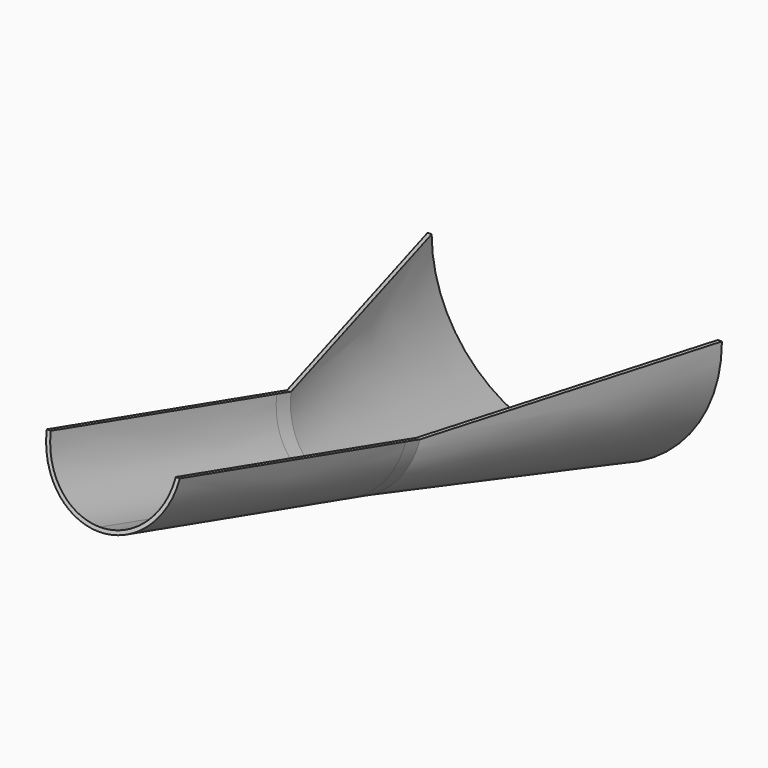
from build123d import *

# Parameters (mm, degrees)
F1_ANGLE      = 180
F3_DEPTH      = 44.6
F3_DEPTH_BACK = 39.8
F4_DEPTH      = 25
F5_DEPTH      = 25
F6_DEPTH      = 152.4


with BuildPart() as f1:
    # F0 (on Top) → F1 (revolve)
    with BuildSketch(Plane.XY):
        Polygon((-31.75, 0), (-29.6666666667, 0), (-74.1166666667, 152.4), (-76.2, 152.4), align=None)
    revolve(axis=Axis((0, 76.2, 0), (0, -1, 0)), revolution_arc=F1_ANGLE)

    # F2 (on Right) → F3 (join, two sides)
    with BuildSketch(Plane.YZ) as f3_sk:
        Polygon((-9.2604166667, -29.0490451389), (0, -31.75), (9.2604166667, 0), (0, 2.7009548611), align=None)
    extrude(amount=F3_DEPTH)
    extrude(f3_sk.sketch, amount=-F3_DEPTH_BACK)

    # F4 (cut): faces of the model
    f4_faces = [f1.faces().sort_by_distance(p)[0] for p in [
        (33.8924298462, 3.5692640267, -19.5125233371),
        (-30.9009295453, 3.1872250967, -20.8223710971),
    ]]
    extrude(f4_faces, amount=-F4_DEPTH, mode=Mode.SUBTRACT)

    # F5 (cut): a face of the model
    f5_faces = [f1.faces().sort_by_distance(p)[0] for p in [
        (0, 5.5929259121, -12.5742540156),
    ]]
    extrude(f5_faces, amount=-F5_DEPTH, mode=Mode.SUBTRACT)

    # F6 (add): a face of the model
    f6_faces = [f1.faces().sort_by_distance(p)[0] for p in [
        (33.4092881944, -0.2139993496, 1.9672428053),
    ]]
    extrude(f6_faces, amount=F6_DEPTH)


solid = f1.part
